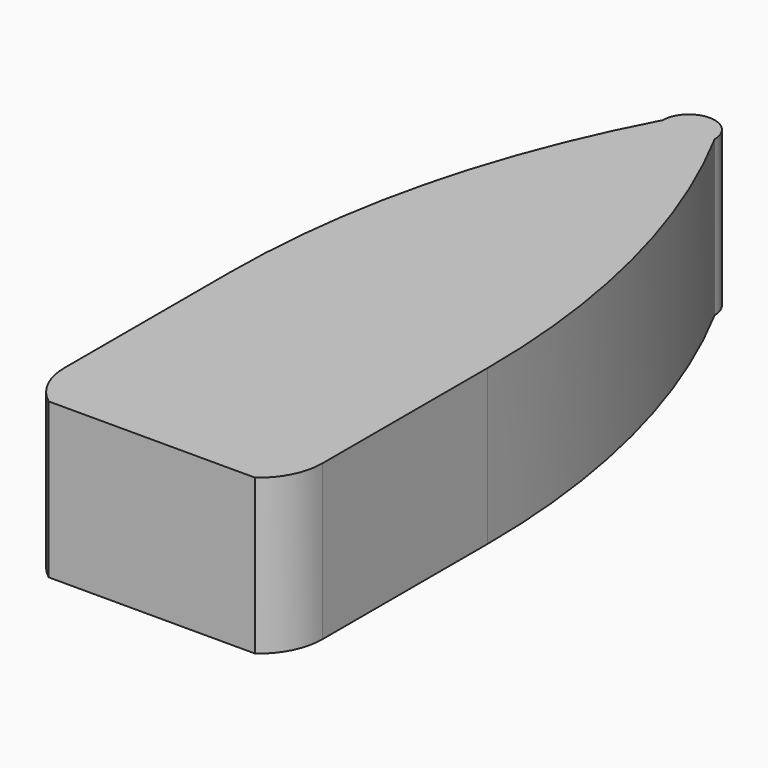
from build123d import *

# Parameters (mm, degrees)
F1_DEPTH = 76.2


# Not quite as in the source:
# - a feature of the source that left no trace in its solid (it failed there, or was rolled back) is left out


with BuildPart() as f1:
    # F0 (on Top) → F1 (new body)
    with BuildSketch(Plane.XY):
        with BuildLine():
            Line((0, 203.2), (0, 0))
            Line((0, 0), (63.5, 0))
            ThreePointArc((63.5, 0), (50.6075315628, 104.7268828907), (12.7, 203.2))
            Line((12.7, 203.2), (0, 203.2))
        make_face()
        with BuildLine():
            Line((-63.5, 0), (0, 0))
            Line((0, 0), (0, 203.2))
            Line((0, 203.2), (-12.7, 203.2))
            ThreePointArc((-12.7, 203.2), (-50.6075315628, 104.7268828907), (-63.5, 0))
        make_face()
        with BuildLine():
            Line((0, 215.9), (0, 203.2))
            Line((0, 203.2), (12.7, 203.2))
            ThreePointArc((12.7, 203.2), (8.9802561211, 212.1802561211), (0, 215.9))
        make_face()
        with BuildLine():
            Line((-12.7, 203.2), (0, 203.2))
            Line((0, 203.2), (0, 215.9))
            ThreePointArc((0, 215.9), (-8.9802561211, 212.1802561211), (-12.7, 203.2))
        make_face()
        with BuildLine():
            Line((0, -127), (0, 0))
            Line((0, 0), (-63.5, 0))
            Line((-63.5, 0), (-63.5, -101.6))
            ThreePointArc((-63.5, -101.6), (-60.1480633142, -115.7990316571), (-50.8, -127))
            Line((-50.8, -127), (0, -127))
        make_face()
        with BuildLine():
            Line((63.5, 0), (0, 0))
            Line((0, 0), (0, -127))
            Line((0, -127), (50.8, -127))
            ThreePointArc((50.8, -127), (60.1480633142, -115.7990316571), (63.5, -101.6))
            Line((63.5, -101.6), (63.5, 0))
        make_face()
    extrude(amount=F1_DEPTH)


solid = f1.part
